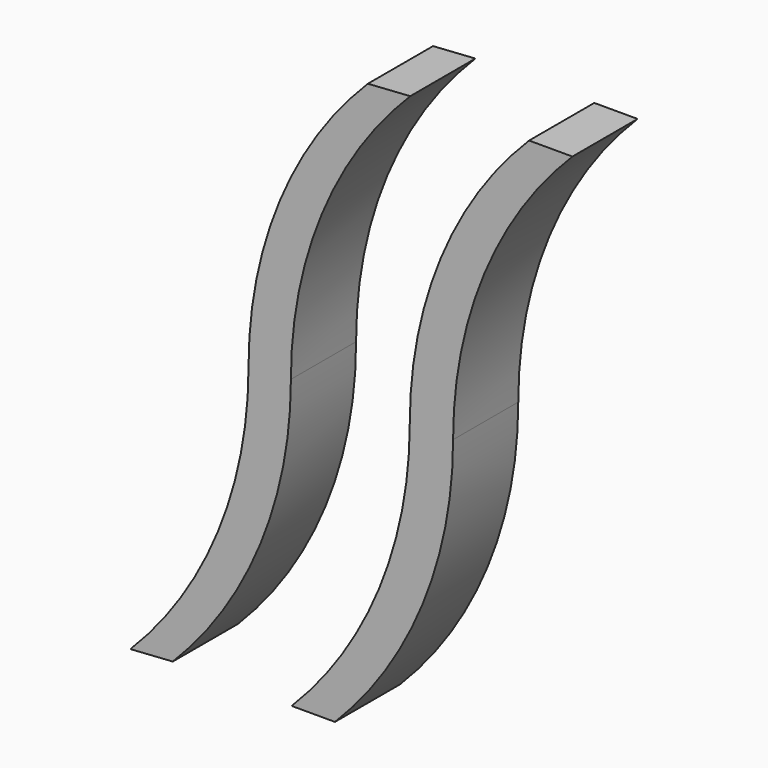
from build123d import *

# Parameters (mm, degrees)
F1_DEPTH = 25.4


# Not quite as in the source:
# - ends of sketch curves that miss each other by under 0.0002 mm in the source are joined


with BuildPart() as f1:
    # F0 (on Front) → F1 (new body)
    with BuildSketch(Plane.XZ):
        with BuildLine():
            Line((-68.8927756, -90.0507216), (-55.6850804, -89.177495))
            ThreePointArc((-55.6850804, -89.177495), (-28.4287580313, -48.1068164863), (-18.8629798, 0.248158))
            ThreePointArc((-18.8629798, 0.248158), (-9.1956804289, 48.8489539104), (18.3344589893, 90.0507192107))
            Line((18.3344589893, 90.0507192107), (5.126736, 89.177495))
            ThreePointArc((5.126736, 89.177495), (-22.4034010289, 47.9757273104), (-32.0707004, -0.6250686))
            ThreePointArc((-32.0707004, -0.6250686), (-41.6364752264, -48.9800348173), (-68.8927756, -90.0507216))
        make_face()
    extrude(amount=F1_DEPTH)


with BuildPart() as f1b:
    # F0 (on Front) → F1, piece 2 (new body)
    with BuildSketch(Plane.XZ):
        with BuildLine():
            ThreePointArc((18.1919626, 0.1251204), (8.6261843687, -48.2298540863), (-18.6301406688, -89.3005299535))
            Line((-18.6301406688, -89.3005299535), (-5.126736, -89.3005326))
            ThreePointArc((-5.126736, -89.3005326), (22.1295863687, -48.2298540863), (31.6953646, 0.1251204))
            ThreePointArc((31.6953646, 0.1251204), (41.3626639711, 48.7259163104), (68.8928033893, 89.9276816107))
            Line((68.8928033893, 89.9276816107), (55.389399, 89.927684))
            ThreePointArc((55.389399, 89.927684), (27.8592619711, 48.7259163104), (18.1919626, 0.1251204))
        make_face()
    extrude(amount=F1_DEPTH)


solid = Compound([f1.part, f1b.part])
